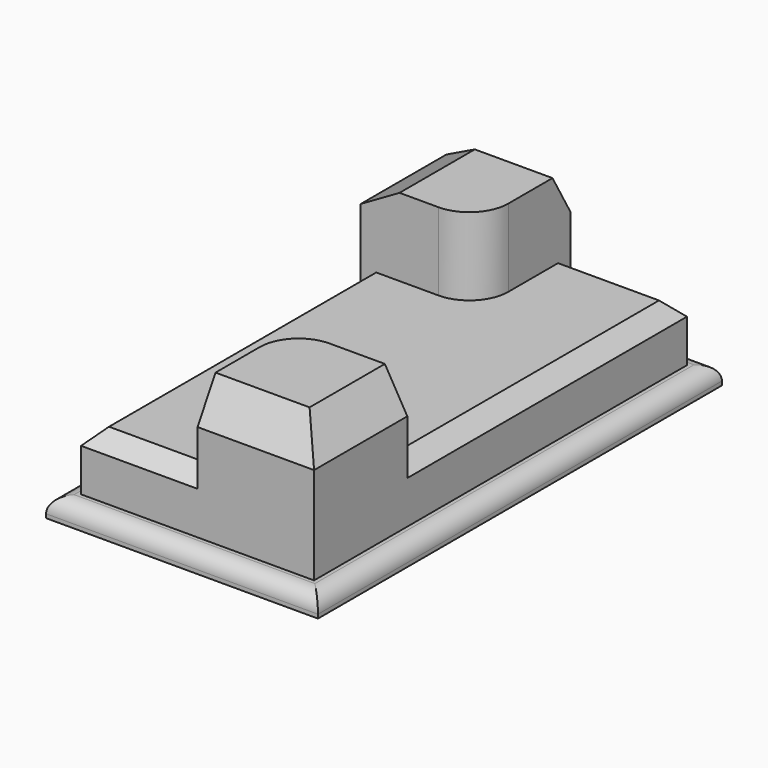
from build123d import *

# Parameters (mm, degrees)
F0_W        = 88.9
F0_H        = 165.1
F1_DEPTH    = 6.35
F2_DEPTH    = 25.4
F3_SIZE     = 5.08
F4_DEPTH    = 50.8
F5_R        = 5.08
F6_C1_SIZE2 = 12.7
F6_C1_SIZE  = 7.3323484187
F6_C2_SIZE2 = 7.3323484187
F6_C2_SIZE  = 12.7
F6_C3_SIZE2 = 7.3323484187
F6_C3_SIZE  = 12.7
F6_C4_SIZE2 = 7.3323484187
F6_C4_SIZE  = 12.7


with BuildPart() as f1:
    # F0 (on Top) → F1 (new body)
    with BuildSketch(Plane.XY):
        Rectangle(F0_W, F0_H)
        Polygon((-38.1, 38.1), (-38.1, 76.2), (0, 76.2), (38.1, 76.2), (38.1, -38.1), (38.1, -76.2), (0, -76.2), (-38.1, -76.2), align=None, mode=Mode.SUBTRACT)
    extrude(amount=F1_DEPTH)

    # F0 (on Top) → F2 (join)
    with BuildSketch(Plane.XY):
        with BuildLine():
            Line((38.1, 76.2), (0, 76.2))
            Line((0, 76.2), (0, 50.8))
            ThreePointArc((0, 50.8), (-3.7197438789, 41.8197438789), (-12.7, 38.1))
            Line((-12.7, 38.1), (-38.1, 38.1))
            Line((-38.1, 38.1), (-38.1, -76.2))
            Line((-38.1, -76.2), (0, -76.2))
            Line((0, -76.2), (0, -50.8))
            ThreePointArc((0, -50.8), (3.7197438789, -41.8197438789), (12.7, -38.1))
            Line((12.7, -38.1), (38.1, -38.1))
            Line((38.1, -38.1), (38.1, 76.2))
        make_face()
    extrude(amount=F2_DEPTH)

    # F3
    f3_edges = [f1.edges().sort_by_distance(p)[0] for p in [
        (-38.1, -19.05, 25.4),
        (-19.05, -76.2, 25.4),
        (38.1, 19.05, 25.4),
        (19.05, 76.2, 25.4),
    ]]
    chamfer(f3_edges, length=F3_SIZE)

    # F0 (on Top) → F4 (join)
    with BuildSketch(Plane.XY):
        with BuildLine():
            Line((38.1, -76.2), (38.1, -38.1))
            Line((38.1, -38.1), (12.7, -38.1))
            ThreePointArc((12.7, -38.1), (3.7197438789, -41.8197438789), (0, -50.8))
            Line((0, -50.8), (0, -76.2))
            Line((0, -76.2), (38.1, -76.2))
        make_face()
        with BuildLine():
            Line((0, 76.2), (-38.1, 76.2))
            Line((-38.1, 76.2), (-38.1, 38.1))
            Line((-38.1, 38.1), (-12.7, 38.1))
            ThreePointArc((-12.7, 38.1), (-3.7197438789, 41.8197438789), (0, 50.8))
            Line((0, 50.8), (0, 76.2))
        make_face()
    extrude(amount=F4_DEPTH)

    # F5
    f5_edges = [f1.edges().sort_by_distance(p)[0] for p in [
        (0, 82.55, 6.35),
        (-44.45, 0, 6.35),
        (0, -82.55, 6.35),
        (44.45, 0, 6.35),
    ]]
    fillet(f5_edges, radius=F5_R)

    # F6: chamfer of 12.7 x 7.3323484187 on 4 edges, made by hand

    # F6_c1
    f6_c1_edges = [f1.edges().sort_by_distance(p)[0] for p in [
        (-38.1, 57.15, 50.8),
    ]]
    f6_c1_side = f1.faces().sort_by_distance((-38.1, 57.15, 50.6533530316))[0]
    chamfer(f6_c1_edges, length=F6_C1_SIZE, length2=F6_C1_SIZE2, reference=f6_c1_side)

    # F6_c2
    f6_c2_edges = [f1.edges().sort_by_distance(p)[0] for p in [
        (-12.7, 76.2, 50.8),
    ]]
    f6_c2_side = f1.faces().sort_by_distance((-12.7, 76.2, 50.6533530316))[0]
    chamfer(f6_c2_edges, length=F6_C2_SIZE, length2=F6_C2_SIZE2, reference=f6_c2_side)

    # F6_c3
    f6_c3_edges = [f1.edges().sort_by_distance(p)[0] for p in [
        (38.1, -57.15, 50.8),
    ]]
    f6_c3_side = f1.faces().sort_by_distance((38.1, -57.15, 50.6533530316))[0]
    chamfer(f6_c3_edges, length=F6_C3_SIZE, length2=F6_C3_SIZE2, reference=f6_c3_side)

    # F6_c4
    f6_c4_edges = [f1.edges().sort_by_distance(p)[0] for p in [
        (15.3838257906, -76.2, 50.8),
    ]]
    f6_c4_side = f1.faces().sort_by_distance((15.3838257906, -76.2, 50.6533530316))[0]
    chamfer(f6_c4_edges, length=F6_C4_SIZE, length2=F6_C4_SIZE2, reference=f6_c4_side)


solid = f1.part
